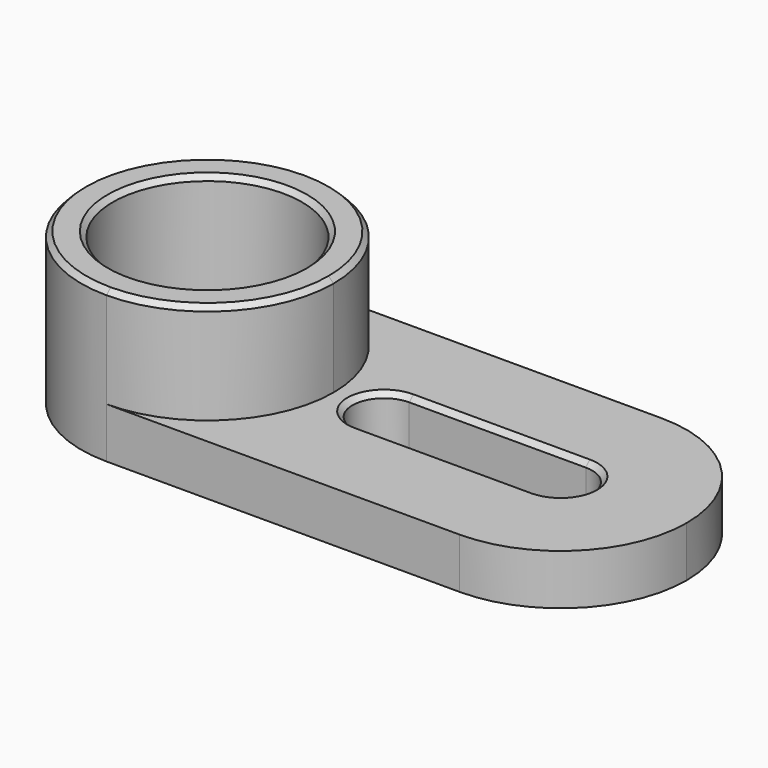
from build123d import *

# Parameters (mm, degrees)
F0_R     = 37.5
F1_DEPTH = 20
F2_DEPTH = 60
F3_SIZE  = 2
F4_SIZE  = 2
F5_SIZE  = 2


# Not quite as in the source:
# - a feature names something its author has since deleted; it is built from what else it names


with BuildPart() as f1:
    # F0 (on Top) → F1 (new body)
    with BuildSketch(Plane.XY):
        with BuildLine():
            ThreePointArc((120, 0), (105.355339, 35.355339), (70, 50))
            ThreePointArc((70, 50), (39.381378, 39.528471), (21.587708, 12.5))
            Line((21.587708, 12.5), (70, 12.5))
            ThreePointArc((70, 12.5), (82.5, 0), (70, -12.5))
            Line((70, -12.5), (21.587708, -12.5))
            ThreePointArc((21.587708, -12.5), (39.381378, -39.528471), (70, -50))
            ThreePointArc((70, -50), (105.355339, -35.355339), (120, 0))
        make_face()
        with BuildLine():
            ThreePointArc((-70, 50), (-34.644661, 35.355339), (-20, 0))
            ThreePointArc((-20, 0), (-34.644661, -35.355339), (-70, -50))
            Line((-70, -50), (70, -50))
            ThreePointArc((70, -50), (39.381378, -39.528471), (21.587708, -12.5))
            Line((21.587708, -12.5), (0, -12.5))
            ThreePointArc((0, -12.5), (-12.5, 0), (0, 12.5))
            Line((0, 12.5), (21.587708, 12.5))
            ThreePointArc((21.587708, 12.5), (39.381378, 39.528471), (70, 50))
            Line((70, 50), (-70, 50))
        make_face()
        with BuildLine():
            ThreePointArc((-70, -50), (-34.644661, -35.355339), (-20, 0))
            ThreePointArc((-20, 0), (-34.644661, 35.355339), (-70, 50))
            ThreePointArc((-70, 50), (-120, 0), (-70, -50))
        make_face()
        with Locations((-70, 0)):
            Circle(F0_R, mode=Mode.SUBTRACT)
    extrude(amount=F1_DEPTH)

    # F0 (on Top) → F2 (join)
    with BuildSketch(Plane.XY):
        with BuildLine():
            ThreePointArc((-70, -50), (-34.644661, -35.355339), (-20, 0))
            ThreePointArc((-20, 0), (-34.644661, 35.355339), (-70, 50))
            ThreePointArc((-70, 50), (-120, 0), (-70, -50))
        make_face()
        with Locations((-70, 0)):
            Circle(F0_R, mode=Mode.SUBTRACT)
    extrude(amount=F2_DEPTH)

    # F3
    f3_edges = [f1.edges().sort_by_distance(p)[0] for p in [
        (-107.5, 0, 60),
        (-70, -50, 60),
    ]]
    chamfer(f3_edges, length=F3_SIZE)

    # F4
    f4_edges = [f1.edges().sort_by_distance(p)[0] for p in [
        (35, 12.5, 20),
    ]]
    chamfer(f4_edges, length=F4_SIZE)

    # F5
    f5_edges = [f1.edges().sort_by_distance(p)[0] for p in [
        (35, -12.5, 0),
        (-107.5, 0, 0),
    ]]
    chamfer(f5_edges, length=F5_SIZE)


solid = f1.part
